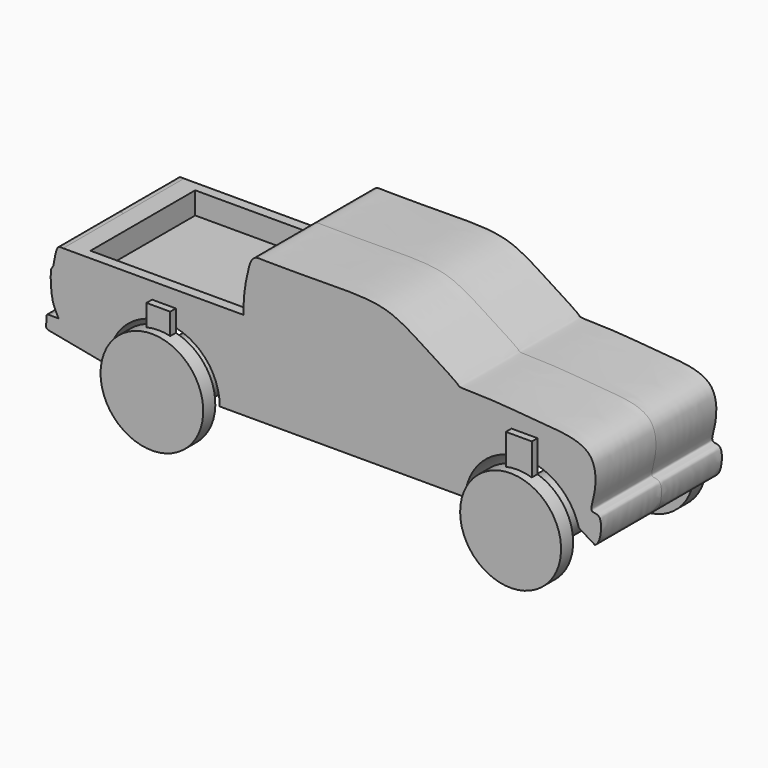
from build123d import *

# Parameters (mm, degrees)
F1_DEPTH  = 19.05
F2_W      = 40.64
F2_H      = 33.02
F3_DEPTH  = 5.588
F4_R      = 12.9540001242
F5_DEPTH  = 3.81
F4_R_2    = 12.7302206493
F7_R      = 7.0441186389
F9_DEPTH  = 40.386
F8_R      = 7.0485
F10_W     = 5.9898644686
F10_H     = 10.2876098827
F11_DEPTH = 1.778
F12_W     = 6.5537057817
F12_H     = 11.1359739676
F13_DEPTH = 1.778


# Not quite as in the source:
# - a feature names something its author has since deleted; it is built from what else it names


with BuildPart() as f1:
    # F0 (on Front) → F1 (new body, symmetric)
    with BuildSketch(Plane.XZ):
        with BuildLine():
            add(Edge.make_bspline(
                [(-69.2842155695, -1.5603305073), (-69.5350025172, -1.5399307664), (-70.1964658552, -1.526121286), (-69.9018841173, -3.0286902092), (-70.3645967063, -4.8077768479), (-69.5958865333, -4.978686168), (-69.2788809538, -5.04994113)],
                knots=[0, 0, 0, 0, 0.1954252336, 0.4695328217, 0.7775236757, 1, 1, 1, 1], degree=3))
            Line((-69.2788809538, -5.04994113), (-54.4446744025, -7.8905327246))
            ThreePointArc((-54.4446744025, -7.8905327246), (-40.3995271772, 6.3133119394), (-26.354379952, -7.8905327246))
            Line((-26.354379952, -7.8905327246), (35.5073921382, -7.8905327246))
            ThreePointArc((35.5073921382, -7.8905327246), (48.7999211019, 5.5232241619), (64.2289370298, -5.3655621596))
            Line((64.2289370298, -5.3655621596), (68.332016468, -7.8905327246))
            add(Edge.make_bspline(
                [(68.332016468, -7.8905327246), (68.7067913051, -7.5679449616), (69.714492426, -6.7005653561), (70.3172984159, -0.4392585426), (66.7802927419, -1.0958089063), (68.4028013282, 2.9762612334), (69.2917253521, 14.2725497335), (53.5065140597, 14.7113305441), (43.8771565321, 16.0310681315), (33.8781446405, 15.9310273294), (33.9330328582, 16.6675611215), (26.0002542616, 21.5508658082), (18.2176068002, 26.7807544456), (11.4548434095, 28.1451041805), (3.6587892983, 28.3191044585), (-14.7558362833, 27.9741795524), (-17.1668552051, 28.3644164723), (-18.5859335818, 27.0949449022), (-19.2248198393, 24.36459907), (-20.2441867929, 19.8982618034), (-20.3211424661, 16.2882279072), (-20.3614756465, 14.3961757421)],
                knots=[0, 0, 0, 0, 0.0298592954, 0.0802861944, 0.110508584, 0.1504361757, 0.217563582, 0.2973555397, 0.3741757692, 0.438561904, 0.4519709004, 0.5165255825, 0.5881373031, 0.6432617714, 0.7085227769, 0.8031750452, 0.8361448558, 0.8632792375, 0.8998543586, 0.9475127428, 1, 1, 1, 1], degree=3))
            Line((-20.3614756465, 14.3961757421), (-65.8321008086, 14.3961757421))
            add(Edge.make_bspline(
                [(-65.8321008086, 14.3961757421), (-66.1119049823, 14.4054631172), (-66.6227405068, 14.4224189798), (-67.2879149417, 14.2751954831), (-67.9931529597, 11.9924706508), (-68.1930622811, 9.4607186493), (-69.0930767314, 9.0286087442), (-68.9238735496, 4.2425680846), (-68.3896505368, 1.0708895061), (-67.4304833389, -0.7146991208), (-66.9762343168, -1.5603305073)],
                knots=[0, 0, 0, 0, 0.0788218688, 0.1439042534, 0.2790854206, 0.4187108143, 0.4966559878, 0.6831908786, 0.8499633496, 1, 1, 1, 1], degree=3))
            Line((-66.9762343168, -1.5603305073), (-69.2842155695, -1.5603305073))
        make_face()
    extrude(amount=F1_DEPTH, both=True)

    # F2 (on face) → F3 (cut)
    with BuildSketch(Plane.XY.offset(14.3961757421)):
        with Locations((-40.6465960781, 0)):
            Rectangle(F2_W, F2_H)
    extrude(amount=-F3_DEPTH, mode=Mode.SUBTRACT)



with BuildPart() as f5:
    # F4 (on face) → F5 (new body)
    with BuildSketch(Plane(origin=(0, 19.05, 0), x_dir=(-1, 0, 0), z_dir=(0, 1, 0))):
        with Locations((40.3995271772, -7.7327218372)):
            Circle(F4_R)
    extrude(amount=F5_DEPTH)


with BuildPart() as f5b:
    # F4 (on face) → F5, piece 2 (new body)
    with BuildSketch(Plane(origin=(0, 19.05, 0), x_dir=(-1, 0, 0), z_dir=(0, 1, 0))):
        with Locations((-50.0800661584, -9.0384282465)):
            Circle(F4_R_2)
    extrude(amount=F5_DEPTH)


with BuildPart() as f6_1:
    # F6: instance of F5
    add(f5.part.mirror(Plane.XZ))


with BuildPart() as f6_2:
    # F6: instance of F5b
    add(f5b.part.mirror(Plane.XZ))


with BuildPart() as f5_1:
    add(f5.part)

    add(f6_1.part)  # F9 merges F6_1
    # F7 (on face) → F9 (join)
    with BuildSketch(Plane(origin=(0, -19.05, 0), x_dir=(-1, 0, 0), z_dir=(0, 1, 0))):
        with Locations((40.3995271772, -7.7327218372)):
            Circle(F7_R)
    extrude(amount=F9_DEPTH)


with BuildPart() as f5b_1:
    add(f5b.part)

    add(f6_2.part)  # F9#2 merges F6_2
    # F8 (on face) → F9, piece 2 (join)
    with BuildSketch(Plane(origin=(0, -19.05, 0), x_dir=(-1, 0, 0), z_dir=(0, 1, 0))):
        with Locations((-50.0800661584, -9.0384282465)):
            Circle(F8_R)
    extrude(amount=F9_DEPTH)


with BuildPart() as f1_1:
    add(f1.part)

    add(f5_1.part)  # F11 merges F5
    # F10 (on face) → F11 (join)
    with BuildSketch(Plane(origin=(0, 19.05, 0), x_dir=(-1, 0, 0), z_dir=(0, 1, 0))):
        with Locations((40.3925478458, 5.1438049413)):
            Rectangle(F10_W, F10_H)
    extrude(amount=F11_DEPTH)


    add(f5b_1.part)  # F13 merges F5b
    # F12 (on face) → F13 (join)
    with BuildSketch(Plane(origin=(0, 19.05, 0), x_dir=(-1, 0, 0), z_dir=(0, 1, 0))):
        with Locations((-50.5348350853, 5.5679869838)):
            Rectangle(F12_W, F12_H)
    extrude(amount=F13_DEPTH)

    # F14: F1 across plane


with BuildPart() as f1_2:
    add(f1_1.part)
    add(f1_1.part.mirror(Plane.XZ))


solid = f1_2.part
